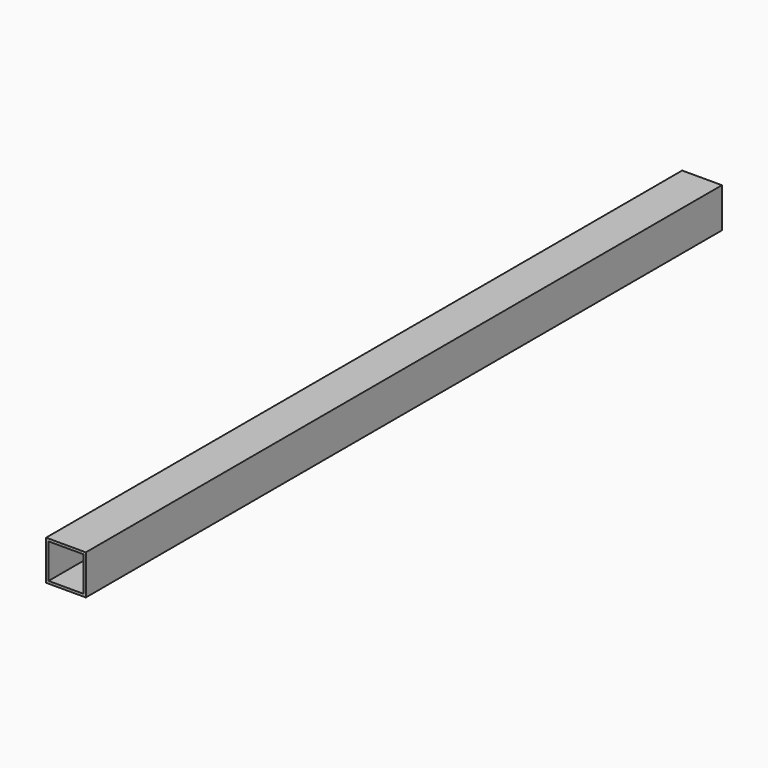
from build123d import *

# Parameters (mm, degrees)
F1_W     = 25.4
F1_H     = 25.4
F1_W_2   = 22.225
F1_H_2   = 22.225
F2_DEPTH = 508


# Not quite as in the source:
# - a variable given as a bare number and used for a length is read in inches; the dataset says mm whatever the document's units were


with BuildPart() as f2:
    # F1 (on Front) → F2 (new body)
    with BuildSketch(Plane.XZ):
        Rectangle(F1_W, F1_H)
        Rectangle(F1_W_2, F1_H_2, mode=Mode.SUBTRACT)
    extrude(amount=F2_DEPTH)


solid = f2.part
